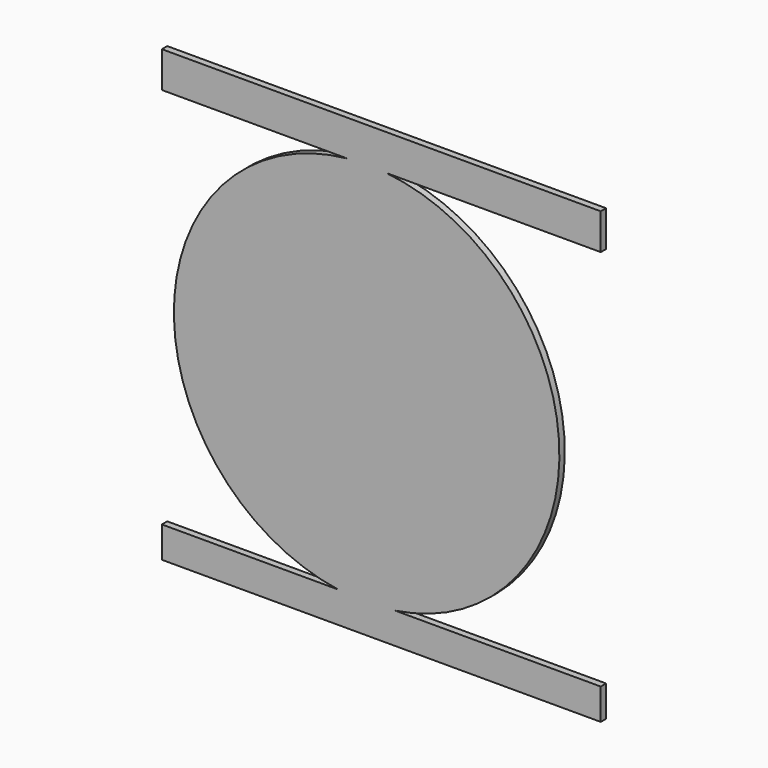
from build123d import *

# Parameters (mm, degrees)
F1_DEPTH = 25.4
F3_DEPTH = 25.4


# Not quite as in the source:
# - the program builds the solid bodies; features that only make, move or delete a surface that nothing else refers to are left out


with BuildPart() as f1:
    # F0 (on Front) → F1 (new body)
    with BuildSketch(Plane.XZ):
        with BuildLine():
            ThreePointArc((-73.432606987, 725.1798510551), (0, 728.8883070439), (73.432606987, 725.1798510551))
            Line((73.432606987, 725.1798510551), (885.1755261421, 725.1798510551))
            Line((885.1755261421, 725.1798510551), (885.1755261421, 861.151099205))
            Line((885.1755261421, 861.151099205), (-774.2805480957, 861.151099205))
            Line((-774.2805480957, 861.151099205), (-774.2805480957, 725.1798510551))
            Line((-774.2805480957, 725.1798510551), (-73.432606987, 725.1798510551))
        make_face()
    extrude(amount=F1_DEPTH)

    # F0 (on Front) → F3 (join)
    with BuildSketch(Plane.XZ):
        with BuildLine():
            ThreePointArc((107.6199000481, -720.8995223045), (552.1417620936, -475.8336250177), (728.8883070439, 0))
            ThreePointArc((728.8883070439, 0), (540.7413118737, 488.7504452974), (73.432606987, 725.1798510551))
            Line((73.432606987, 725.1798510551), (-73.432606987, 725.1798510551))
            ThreePointArc((-73.432606987, 725.1798510551), (-728.6846993659, 17.2271023467), (-107.6199000481, -720.8995223045))
            Line((-107.6199000481, -720.8995223045), (107.6199000481, -720.8995223045))
        make_face()
        with BuildLine():
            Line((-73.432606987, 725.1798510551), (73.432606987, 725.1798510551))
            ThreePointArc((73.432606987, 725.1798510551), (0, 728.8883070439), (-73.432606987, 725.1798510551))
        make_face()
        with BuildLine():
            ThreePointArc((-73.432606987, 725.1798510551), (0, 728.8883070439), (73.432606987, 725.1798510551))
            Line((73.432606987, 725.1798510551), (885.1755261421, 725.1798510551))
            Line((885.1755261421, 725.1798510551), (885.1755261421, 861.151099205))
            Line((885.1755261421, 861.151099205), (-774.2805480957, 861.151099205))
            Line((-774.2805480957, 861.151099205), (-774.2805480957, 725.1798510551))
            Line((-774.2805480957, 725.1798510551), (-73.432606987, 725.1798510551))
        make_face()
        with BuildLine():
            Line((885.1755261421, -720.8995223045), (107.6199000481, -720.8995223045))
            ThreePointArc((107.6199000481, -720.8995223045), (0, -728.8883070439), (-107.6199000481, -720.8995223045))
            Line((-107.6199000481, -720.8995223045), (-774.2805480957, -720.8995223045))
            Line((-774.2805480957, -720.8995223045), (-774.2805480957, -838.6484384537))
            Line((-774.2805480957, -838.6484384537), (885.1755261421, -838.6484384537))
            Line((885.1755261421, -838.6484384537), (885.1755261421, -720.8995223045))
        make_face()
        with BuildLine():
            ThreePointArc((-107.6199000481, -720.8995223045), (0, -728.8883070439), (107.6199000481, -720.8995223045))
            Line((107.6199000481, -720.8995223045), (-107.6199000481, -720.8995223045))
        make_face()
    extrude(amount=F3_DEPTH)


solid = f1.part
